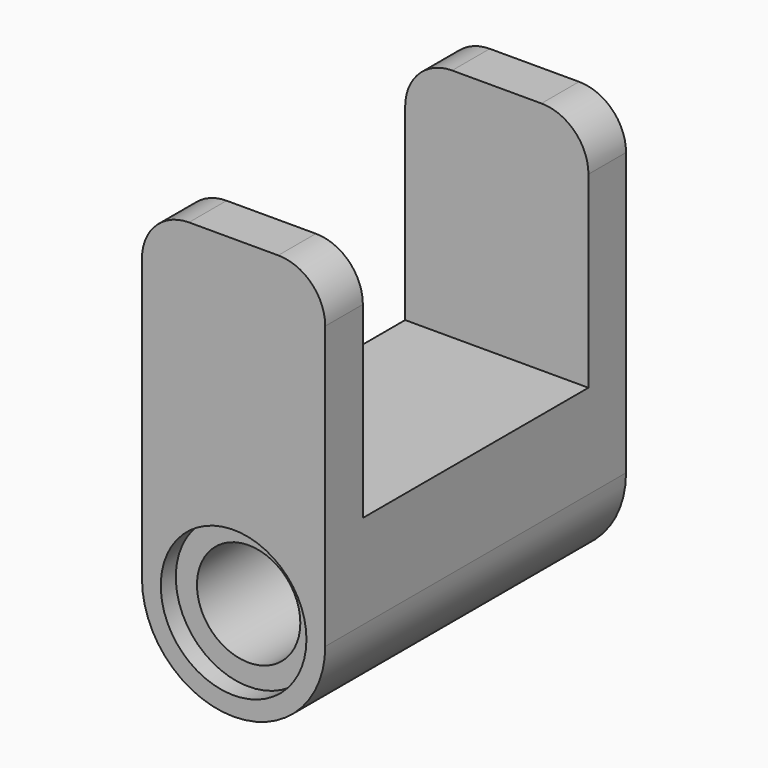
from build123d import *

# Parameters (mm, degrees)
F2_R     = 3.1
F2_R_2   = 2.2
F4_DEPTH = 8
F3_W     = 12
F3_H     = 10
F5_DEPTH = 12.5
F6_R     = 2
F7_DEPTH = 0.8


# Not quite as in the source:
# - the program builds the solid bodies; features that only make, move or delete a surface that nothing else refers to are left out


with BuildPart() as f4:
    # F2 (on Front) → F4 (new body, symmetric)
    with BuildSketch(Plane.XZ):
        with BuildLine():
            Line((3.8994949366, 10), (-3.8994949366, 10))
            Line((-3.8994949366, 10), (-3.8994949366, -4))
            ThreePointArc((-3.8994949366, -4), (0, -7.8994949366), (3.8994949366, -4))
            Line((3.8994949366, -4), (3.8994949366, 10))
        make_face()
        with Locations((0, -4)):
            Circle(F2_R, mode=Mode.SUBTRACT)
        with Locations((0, -4)):
            Circle(F2_R)
        with Locations((0, -4)):
            Circle(F2_R_2, mode=Mode.SUBTRACT)
    extrude(amount=F4_DEPTH, both=True)

    # F3 (on Right) → F5 (cut, symmetric)
    with BuildSketch(Plane.YZ):
        with Locations((0, 5)):
            Rectangle(F3_W, F3_H)
    extrude(amount=F5_DEPTH, both=True, mode=Mode.SUBTRACT)

    # F6
    f6_edges = [f4.edges().sort_by_distance(p)[0] for p in [
        (-3.899495, -7, 10),
        (3.899495, -7, 10),
        (3.899495, 7, 10),
        (-3.899495, 7, 10),
    ]]
    fillet(f6_edges, radius=F6_R)


with BuildPart() as f7:
    # F2 (on Front) → F7 (new body)
    with BuildSketch(Plane.XZ):
        with Locations((0, -4)):
            Circle(F2_R)
        with Locations((0, -4)):
            Circle(F2_R_2, mode=Mode.SUBTRACT)
    extrude(amount=F7_DEPTH)


with BuildPart() as f7_1:
    # F8: moved
    add(f7.part.moved(Location((0, 8, 0))))


with BuildPart() as f9_1:
    # F9: instance of F7
    add(f7_1.part.mirror(Plane.XZ))


with BuildPart() as f4_1:
    add(f4.part)

    # F10: cut F7, F9_1
    add(f7_1.part, mode=Mode.SUBTRACT)
    add(f9_1.part, mode=Mode.SUBTRACT)


solid = f4_1.part
